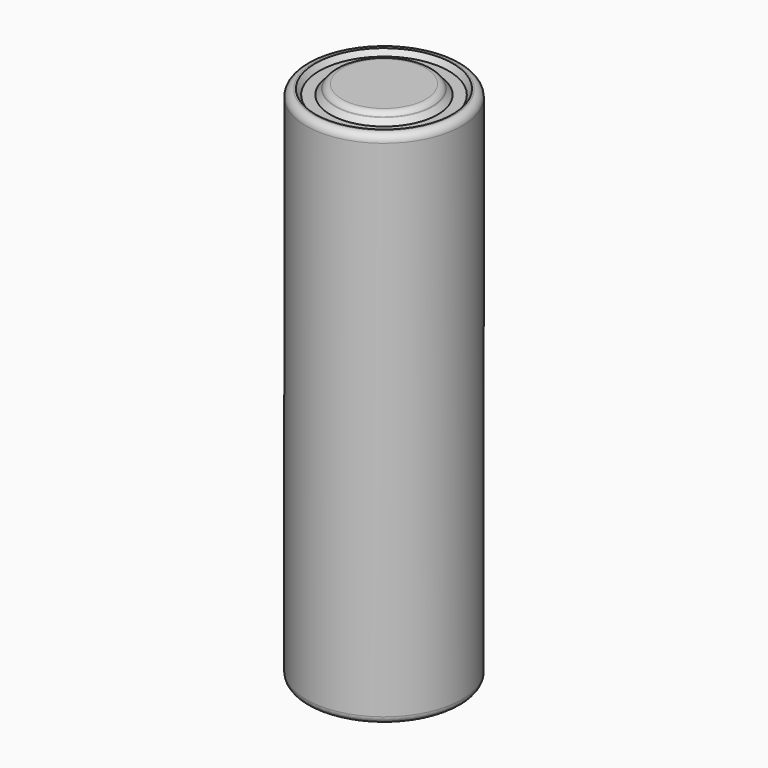
from build123d import *

# Parameters (mm, degrees)
F2_R = 1


# Not quite as in the source:
# - two fillets or chamfers of one size are made in one step


with BuildPart() as f1:
    # F0 (on Front) → F1 (revolve)
    with BuildSketch(Plane.XZ):
        Polygon((-10.4996741857, -0.0827163458), (0, 0), (0, 69.9172836542), (0, 70.5213546753), (-6.2381645857, 70.5213546753), (-6.5643620988, 69.9172836542), (-7.2255664847, 69.2085400224), (-8.7180831586, 69.2085400224), (-9.2690859436, 69.9172836542), (-10.4996741857, 69.9172836542), align=None)
    revolve(axis=Axis((0, 0, 34.9586418271), (0, 0, 1)))

    # F2
    f2_edges = [f1.edges().sort_by_distance(p)[0] for p in [
        (10.499674, 0, -0.082716),
        (6.238165, 0, 70.521355),
        (10.499674, 0, 69.917284),
    ]]
    fillet(f2_edges, radius=F2_R)


solid = f1.part
